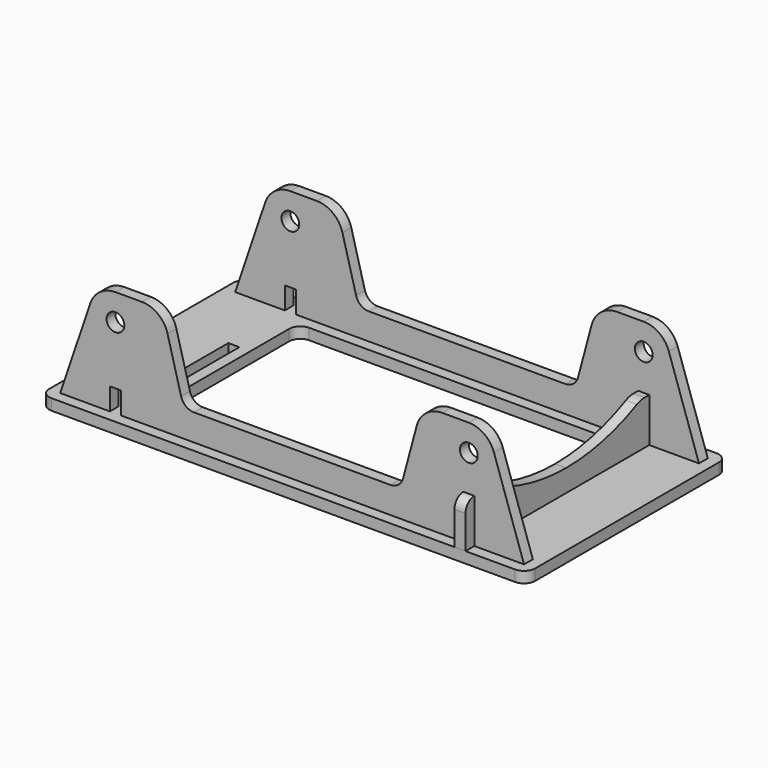
from build123d import *

# Parameters (mm, degrees)
F0_R       = 4.025
F1_DEPTH   = 5
F2_SIZE2   = 2.5
F2_SIZE    = 0.5
F2_2_SIZE2 = 2.5
F2_2_SIZE  = 0.5
F3_SIZE2   = 0.5
F3_SIZE    = 2.5
F5_W       = 30
F5_H       = 5
F6_DEPTH   = 5
F8_DEPTH   = 5
F9_R       = 4.99999
F10_R      = 10
F11_SIZE2  = 2.5
F11_SIZE   = 0.5


# Not quite as in the source:
# - a fillet or chamfer is up to 0.001 mm smaller than in the source, because OpenCascade refuses the exact size


with BuildPart() as f1:
    # F0 (on Front) → F1 (new body)
    with BuildSketch(Plane.XZ):
        with BuildLine():
            Line((-91.3645840485, 40.2173871719), (-105, 0))
            Line((-105, 0), (-82.5, 0))
            Line((-82.5, 0), (-82.5, 10))
            Line((-82.5, 10), (-77.5, 10))
            Line((-77.5, 10), (-77.5, 0))
            Line((-77.5, 0), (-67.5, 0))
            Line((-67.5, 0), (-67.5, -5))
            Line((-67.5, -5), (-37.5, -5))
            Line((-37.5, -5), (-37.5, 0))
            Line((-37.5, 0), (0, 0))
            Line((0, 0), (37.5, 0))
            Line((37.5, 0), (37.5, -5))
            Line((37.5, -5), (67.5, -5))
            Line((67.5, -5), (67.5, 0))
            Line((67.5, 0), (77.5, 0))
            Line((77.5, 0), (77.5, 10))
            Line((77.5, 10), (82.5, 10))
            Line((82.5, 10), (82.5, 0))
            Line((82.5, 0), (105, 0))
            Line((105, 0), (91.3645840485, 40.2173871719))
            ThreePointArc((91.3645840485, 40.2173871719), (86.9915318027, 46.1171771665), (80, 48.3643066634))
            Line((80, 48.3643066634), (68, 48.3643066634))
            ThreePointArc((68, 48.3643066634), (60.6948628519, 45.8845467469), (56.4088900845, 39.4701352046))
            Line((56.4088900845, 39.4701352046), (50.2398825703, 16.4470857294))
            ThreePointArc((50.2398825703, 16.4470857294), (48.0968961867, 13.2398799583), (44.4443276126, 12))
            Line((44.4443276126, 12), (0, 12))
            Line((0, 12), (-44.4443276126, 12))
            ThreePointArc((-44.4443276126, 12), (-48.0968961867, 13.2398799583), (-50.2398825703, 16.4470857294))
            Line((-50.2398825703, 16.4470857294), (-56.4088900845, 39.4701352046))
            ThreePointArc((-56.4088900845, 39.4701352046), (-60.6948628519, 45.8845467469), (-68, 48.3643066634))
            Line((-68, 48.3643066634), (-80, 48.3643066634))
            ThreePointArc((-80, 48.3643066634), (-86.9915318027, 46.1171771665), (-91.3645840485, 40.2173871719))
        make_face()
        with Locations((-80, 36.3643066634)):
            Circle(F0_R, mode=Mode.SUBTRACT)
        with Locations((80, 36.3643066634)):
            Circle(F0_R, mode=Mode.SUBTRACT)
    extrude(amount=F1_DEPTH)

    # F2
    f2_edges = [f1.edges().sort_by_distance(p)[0] for p in [
        (-67.5, -2.5, -5),
        (-37.5, -2.5, -5),
    ]]
    f2_side = f1.faces().sort_by_distance((-52.5, -2.5, -5))[0]
    chamfer(f2_edges, length=F2_SIZE, length2=F2_SIZE2, reference=f2_side)

    # F2#2
    f2_2_edges = [f1.edges().sort_by_distance(p)[0] for p in [
        (37.5, -2.5, -5),
    ]]
    f2_2_side = f1.faces().sort_by_distance((52.5, -2.5, -5))[0]
    chamfer(f2_2_edges, length=F2_2_SIZE, length2=F2_2_SIZE2, reference=f2_2_side)

    # F3
    f3_edges = [f1.edges().sort_by_distance(p)[0] for p in [
        (67.5, -2.5, -5),
    ]]
    f3_side = f1.faces().sort_by_distance((67.5, -2.5, -2.5))[0]
    chamfer(f3_edges, length=F3_SIZE, length2=F3_SIZE2, reference=f3_side)


with BuildPart() as f4_1:
    # F4: copy of F1
    add(f1.part.moved(Location((0, 99, 0))))


with BuildPart() as f6:
    # F5 (on face) → F6 (new body)
    with BuildSketch(Plane(origin=(0, 0, 0), x_dir=(1, 0, 0), z_dir=(0, 0, -1))):
        with BuildLine():
            Line((105, 10), (0, 10))
            Line((0, 10), (-105, 10))
            ThreePointArc((-105, 10), (-108.5355339059, 8.5355339059), (-110, 5))
            Line((-110, 5), (-110, -47))
            Line((-110, -47), (-110, -99))
            ThreePointArc((-110, -99), (-108.5355339059, -102.5355339059), (-105, -104))
            Line((-105, -104), (0, -104))
            Line((0, -104), (105, -104))
            ThreePointArc((105, -104), (108.5355339059, -102.5355339059), (110, -99))
            Line((110, -99), (110, -47))
            Line((110, -47), (110, 5))
            ThreePointArc((110, 5), (108.5355339059, 8.5355339059), (105, 10))
        make_face()
        with Locations((-52.5, -96.5)):
            Rectangle(F5_W, F5_H, mode=Mode.SUBTRACT)
        with Locations((52.5, -96.5)):
            Rectangle(F5_W, F5_H, mode=Mode.SUBTRACT)
        Polygon((-77.5, -32), (-77.5, -47), (-77.5, -62), (-82.5, -62), (-82.5, -47), (-82.5, -32), align=None, mode=Mode.SUBTRACT)
        with Locations((-52.5, 2.5)):
            Rectangle(F5_W, F5_H, mode=Mode.SUBTRACT)
        with BuildLine():
            Line((-72.5, -84), (-72.5, -47))
            Line((-72.5, -47), (-72.5, -10))
            ThreePointArc((-72.5, -10), (-71.0355339059, -6.4644660941), (-67.5, -5))
            Line((-67.5, -5), (0, -5))
            Line((0, -5), (67.5, -5))
            ThreePointArc((67.5, -5), (71.0355339059, -6.4644660941), (72.5, -10))
            Line((72.5, -10), (72.5, -47))
            Line((72.5, -47), (72.5, -84))
            ThreePointArc((72.5, -84), (71.0355339059, -87.5355339059), (67.5, -89))
            Line((67.5, -89), (0, -89))
            Line((0, -89), (-67.5, -89))
            ThreePointArc((-67.5, -89), (-71.0355339059, -87.5355339059), (-72.5, -84))
        make_face(mode=Mode.SUBTRACT)
        Polygon((77.5, -62), (77.5, -47), (77.5, -32), (82.5, -32), (82.5, -47), (82.5, -62), align=None, mode=Mode.SUBTRACT)
        with Locations((52.5, 2.5)):
            Rectangle(F5_W, F5_H, mode=Mode.SUBTRACT)
    extrude(amount=F6_DEPTH)


with BuildPart() as f8:
    # F7 (on face) → F8 (new body)
    with BuildSketch(Plane.YZ.offset(77.5)):
        with BuildLine():
            Line((0, 10), (-5, 10))
            Line((-5, 10), (-5, 20))
            Line((-5, 20), (-10, 20))
            Line((-10, 20), (-10, 0))
            Line((-10, 0), (32, 0))
            Line((32, 0), (32, -5))
            Line((32, -5), (62, -5))
            Line((62, -5), (62, 0))
            Line((62, 0), (104, 0))
            Line((104, 0), (104, 20))
            Line((104, 20), (99, 20))
            Line((99, 20), (99, 10))
            Line((99, 10), (94, 10))
            Line((94, 10), (94, 20))
            Line((94, 20), (89, 20))
            ThreePointArc((89, 20), (68.5870331449, 12.5344607913), (47, 10))
            ThreePointArc((47, 10), (25.4129668551, 12.5344607913), (5, 20))
            Line((5, 20), (0, 20))
            Line((0, 20), (0, 10))
        make_face()
    extrude(amount=F8_DEPTH)

    # F9 (radius 5 in the source; OpenCascade refuses exactly that, so slightly less here)
    f9_edges = [f8.edges().sort_by_distance(p)[0] for p in [
        (80, -10, 20),
        (80, 104, 20),
    ]]
    fillet(f9_edges, radius=F9_R)

    # F10
    f10_edges = [f8.edges().sort_by_distance(p)[0] for p in [
        (80, 5, 20),
        (80, 89, 20),
    ]]
    fillet(f10_edges, radius=F10_R)

    # F11
    f11_edges = [f8.edges().sort_by_distance(p)[0] for p in [
        (80, 32, -5),
        (80, 62, -5),
    ]]
    f11_side = f8.faces().sort_by_distance((80, 47, -5))[0]
    chamfer(f11_edges, length=F11_SIZE, length2=F11_SIZE2, reference=f11_side)


solid = Compound([f1.part, f4_1.part, f6.part, f8.part])
